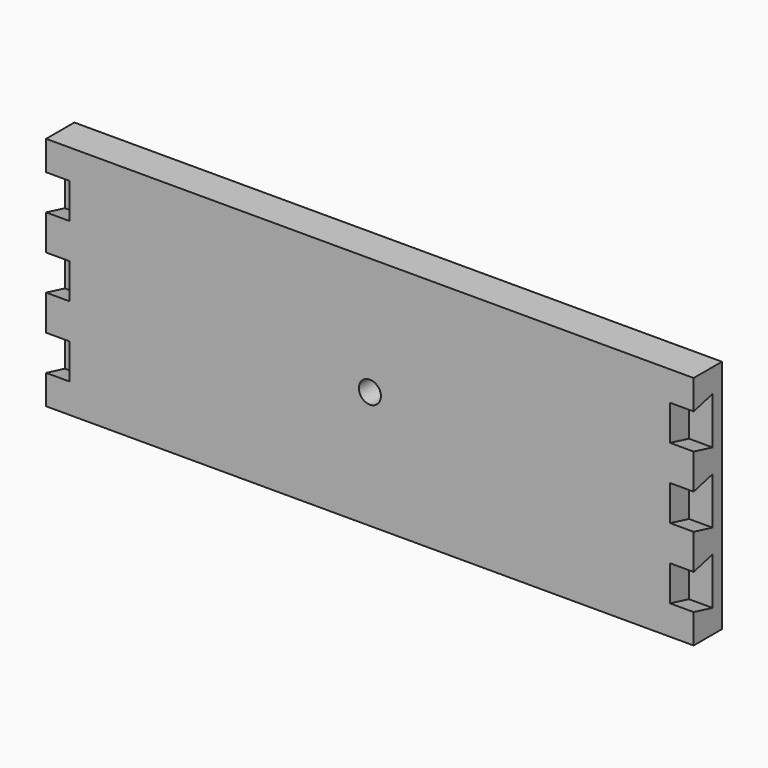
from build123d import *

# Parameters (mm, degrees)
F0_W     = 349.25
F0_H     = 127
F1_DEPTH = 19.05
F3_DEPTH = 12.7
F4_D     = 11.90625
F4_DEPTH = 34.925
F4_TIP   = 3.5769983726


# Not quite as in the source:
# - a pattern or mirror of a feature is missing from the dataset's text; its kind, count and spacing are read off the source's solid


with BuildPart() as f1:
    # F0 (on Front) → F1 (new body)
    with BuildSketch(Plane.XZ):
        Rectangle(F0_W, F0_H)
    extrude(amount=F1_DEPTH)

    # F2 (on face) → F3 (cut)
    with BuildSketch(Plane(origin=(-174.625, 0, 0), x_dir=(0, -1, 0), z_dir=(-1, 0, 0))):
        Polygon((19.05, -47.625), (19.05, -28.575), (6.35, -25.4085343639), (6.35, -50.7914656361), align=None)
        Polygon((19.05, -9.525), (19.05, 9.525), (6.35, 12.6914656361), (6.35, -12.6914656361), align=None)
        Polygon((19.05, 28.575), (19.05, 47.625), (6.35, 50.7914656361), (6.35, 25.4085343639), align=None)
    f3 = extrude(amount=-F3_DEPTH, mode=Mode.SUBTRACT)

    # F3_copies: F3 across plane
    add(f3.mirror(Plane(origin=(0, 0, 0), x_dir=(0, 0, 1), z_dir=(1, 0, 0))), mode=Mode.SUBTRACT)

    # F4
    with Locations(Plane(origin=(0, 0, 0), x_dir=(1, 0, 0), z_dir=(0, 1, 0))):
        with Locations((0, 0)):
            Hole(F4_D / 2, depth=F4_DEPTH)
            with Locations((0, 0, -(F4_DEPTH + F4_TIP / 2))):  # 118° drill point
                Cone(0, F4_D / 2, F4_TIP, mode=Mode.SUBTRACT)


solid = f1.part
